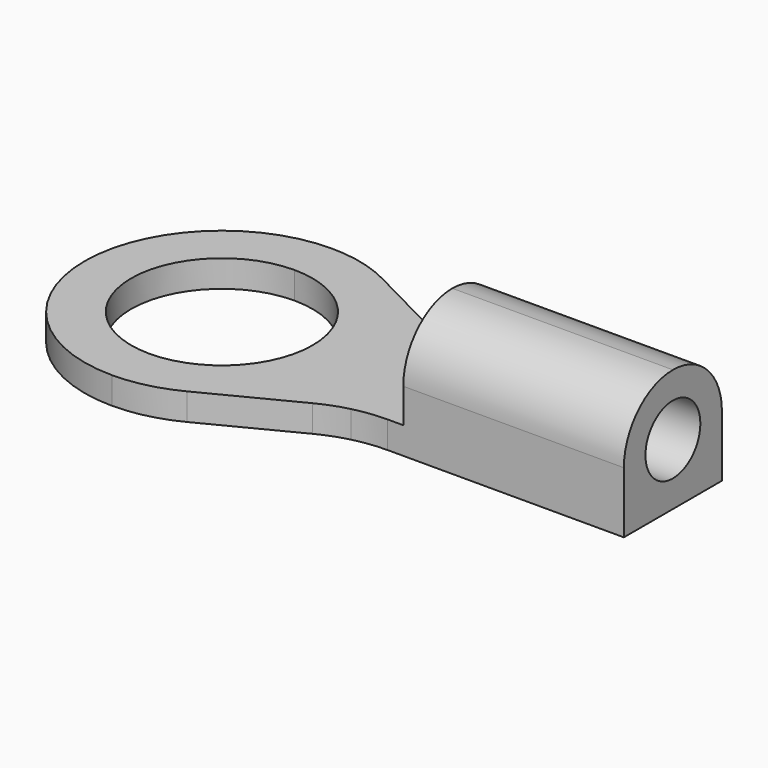
from build123d import *

# Parameters (mm, degrees)
F1_DEPTH = 0.55
F2_W     = 4.5
F2_H     = 2.5
F3_DEPTH = 1.95
F4_R     = 1.24999
F5_R     = 0.7
F6_DEPTH = 25


# Not quite as in the source:
# - a fillet or chamfer is up to 0.001 mm smaller than in the source, because OpenCascade refuses the exact size


with BuildPart() as f1:
    # F0 (on Top) → F1 (new body)
    with BuildSketch(Plane.XY):
        with BuildLine():
            Line((7.1757397782, 1.55), (12, 1.55))
            Line((12, 1.55), (12, 4.05))
            Line((12, 4.05), (7.1757397782, 4.05))
            ThreePointArc((7.1757397782, 4.05), (6.8353451552, 4.0707678217), (6.5, 4.1327632138))
            ThreePointArc((6.5, 4.1327632138), (6.1928359056, 4.2281876541), (5.8986420809, 4.3582091838))
            Line((5.8986420809, 4.3582091838), (4.0770976972, 5.2917908162))
            ThreePointArc((4.0770976972, 5.2917908162), (3.4568811592, 5.5218572965), (2.8, 5.6))
            Line((2.8, 5.6), (2.8, 4.65))
            ThreePointArc((2.8, 4.65), (4.1081475452, 4.1081475452), (4.65, 2.8))
            ThreePointArc((4.65, 2.8), (4.1081475452, 1.4918524548), (2.8, 0.95))
            Line((2.8, 0.95), (2.8, 0))
            ThreePointArc((2.8, 0), (3.4568811592, 0.0781427035), (4.0770976972, 0.3082091838))
            Line((4.0770976972, 0.3082091838), (5.8986420809, 1.2417908162))
            ThreePointArc((5.8986420809, 1.2417908162), (6.1928359056, 1.3718123459), (6.5, 1.4672367862))
            ThreePointArc((6.5, 1.4672367862), (6.8353451552, 1.5292321783), (7.1757397782, 1.55))
        make_face()
        with BuildLine():
            ThreePointArc((0, 2.8), (0.8201010127, 0.8201010127), (2.8, 0))
            Line((2.8, 0), (2.8, 0.95))
            ThreePointArc((2.8, 0.95), (0.95, 2.8), (2.8, 4.65))
            Line((2.8, 4.65), (2.8, 5.6))
            ThreePointArc((2.8, 5.6), (0.8201010127, 4.7798989873), (0, 2.8))
        make_face()
    extrude(amount=F1_DEPTH)

    # F2 (on face) → F3 (join)
    with BuildSketch(Plane.XY.offset(0.55)):
        with Locations((9.75, 2.8)):
            Rectangle(F2_W, F2_H)
    extrude(amount=F3_DEPTH)

    # F4 (radius 1.25 in the source; OpenCascade refuses exactly that, so slightly less here)
    f4_edges = [f1.edges().sort_by_distance(p)[0] for p in [
        (9.75, 4.05, 2.5),
        (9.75, 1.55, 2.5),
    ]]
    fillet(f4_edges, radius=F4_R)

    # F5 (on face) → F6 (cut)
    with BuildSketch(Plane.YZ.offset(12)):
        with Locations((2.8, 1.25)):
            Circle(F5_R)
    extrude(amount=-F6_DEPTH, mode=Mode.SUBTRACT)


solid = f1.part
